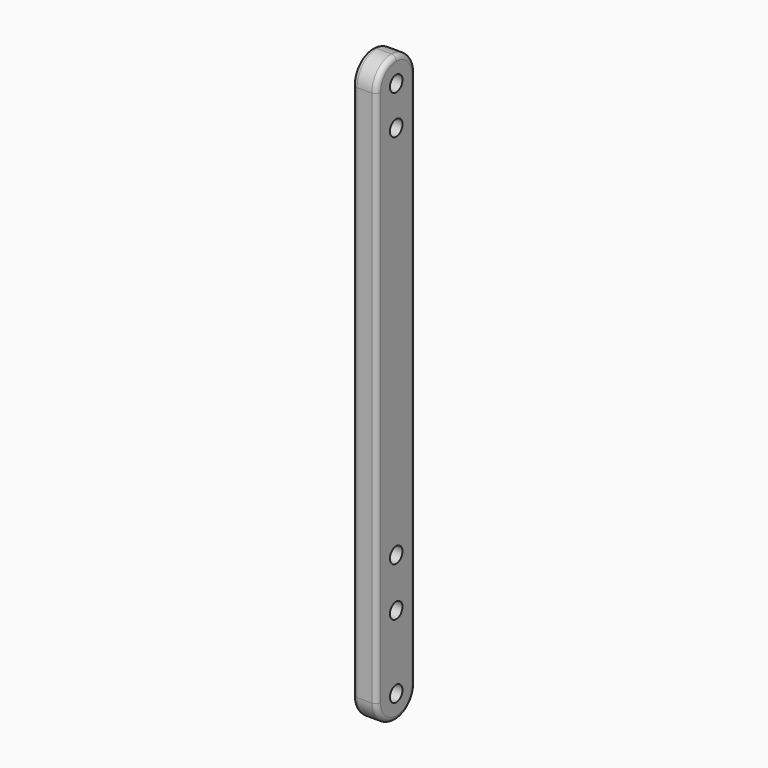
from build123d import *

# Parameters (mm, degrees)
F0_W     = 10
F0_H     = 120
F0_R     = 1.6
F1_DEPTH = 5
F2_R     = 4.99999
F3_R     = 1


# Not quite as in the source:
# - a fillet or chamfer is up to 0.001 mm smaller than in the source, because OpenCascade refuses the exact size


with BuildPart() as f1:
    # F0 (on Right) → F1 (new body)
    with BuildSketch(Plane.YZ):
        with Locations((0, 60)):
            Rectangle(F0_W, F0_H)
        with Locations((0, 5)):
            Circle(F0_R, mode=Mode.SUBTRACT)
        with Locations((0, 20)):
            Circle(F0_R, mode=Mode.SUBTRACT)
        with Locations((0, 30)):
            Circle(F0_R, mode=Mode.SUBTRACT)
        with Locations((0, 107)):
            Circle(F0_R, mode=Mode.SUBTRACT)
        with Locations((0, 115)):
            Circle(F0_R, mode=Mode.SUBTRACT)
    extrude(amount=F1_DEPTH)

    # F2 (radius 5 in the source; OpenCascade refuses exactly that, so slightly less here)
    f2_edges = [f1.edges().sort_by_distance(p)[0] for p in [
        (2.5, 5, 0),
        (2.5, -5, 0),
        (2.5, 5, 120),
        (2.5, -5, 120),
    ]]
    fillet(f2_edges, radius=F2_R)

    # F3
    f3_edges = [f1.edges().sort_by_distance(p)[0] for p in [
        (5, -3.535537, 118.535537),
        (0, 5, 60),
    ]]
    fillet(f3_edges, radius=F3_R)


solid = f1.part
